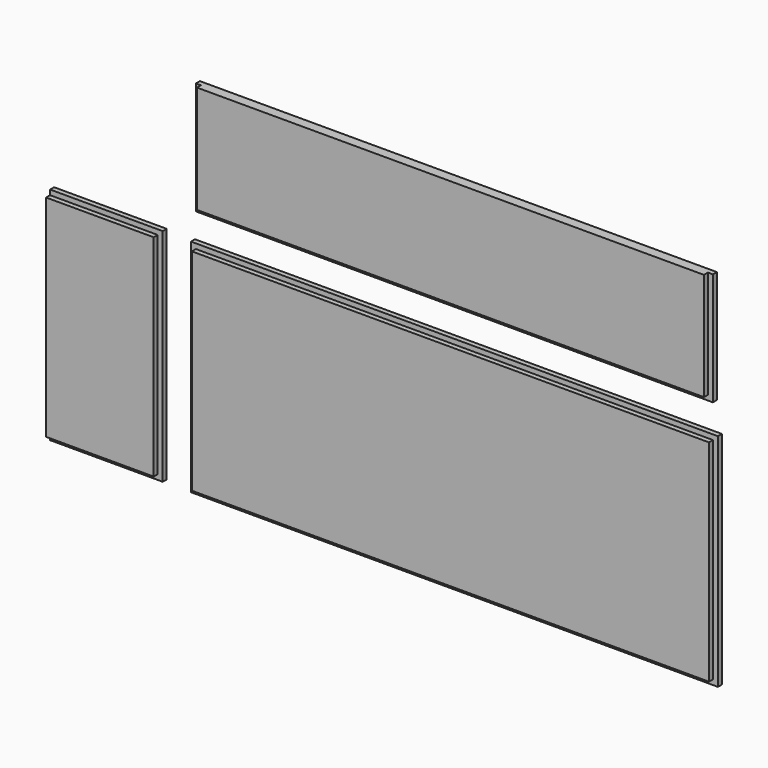
from build123d import *

# Parameters (mm, degrees)
F1_W     = 914.4
F1_H     = 194.183
F2_DEPTH = 18.034
F1_W_2   = 932.434
F1_H_2   = 379.984
F1_W_3   = 194.183
F1_H_3   = 9.017
F3_DEPTH = 9.017
F1_W_4   = 950.468
F1_H_4   = 398.018
F1_W_5   = 9.017


# Not quite as in the source:
# - a variable given as a bare number and used for a length is read in inches; the dataset says mm whatever the document's units were


with BuildPart() as f2:
    # F1 (on Front) → F2 (new body)
    with BuildSketch(Plane.XZ):
        with Locations((0, 355.9175)):
            Rectangle(F1_W, F1_H)
    extrude(amount=F2_DEPTH)

    # F1 (on Front) → F3 (join)
    with BuildSketch(Plane.XZ):
        Polygon((-466.217, 249.809), (-457.2, 249.809), (-457.2, 258.826), (-457.2, 453.009), (-466.217, 453.009), align=None)
        Polygon((457.2, 249.809), (466.217, 249.809), (466.217, 453.009), (457.2, 453.009), (457.2, 258.826), align=None)
        with Locations((0, 254.3175)):
            Rectangle(F1_W, F1_H_3)
    extrude(amount=F3_DEPTH)


with BuildPart() as f2b:
    # F1 (on Front) → F2, piece 2 (new body)
    with BuildSketch(Plane.XZ):
        Rectangle(F1_W_2, F1_H_2)
    extrude(amount=F2_DEPTH)

    # F1 (on Front) → F3, piece 2 (join)
    with BuildSketch(Plane.XZ):
        Rectangle(F1_W_4, F1_H_4)
        Rectangle(F1_W_2, F1_H_2, mode=Mode.SUBTRACT)
    extrude(amount=F3_DEPTH)


with BuildPart() as f2c:
    # F1 (on Front) → F2, piece 3 (new body)
    with BuildSketch(Plane.XZ):
        with Locations((-632.1425, 0)):
            Rectangle(F1_W_3, F1_H_2)
    extrude(amount=F2_DEPTH)

    # F1 (on Front) → F3, piece 3 (join)
    with BuildSketch(Plane.XZ):
        Polygon((-526.034, 189.992), (-526.034, 199.009), (-729.234, 199.009), (-729.234, 189.992), (-535.051, 189.992), align=None)
        with Locations((-530.5425, 0)):
            Rectangle(F1_W_5, F1_H_2)
        Polygon((-526.034, -199.009), (-526.034, -189.992), (-535.051, -189.992), (-729.234, -189.992), (-729.234, -199.009), align=None)
    extrude(amount=F3_DEPTH)


solid = Compound([f2.part, f2b.part, f2c.part])
